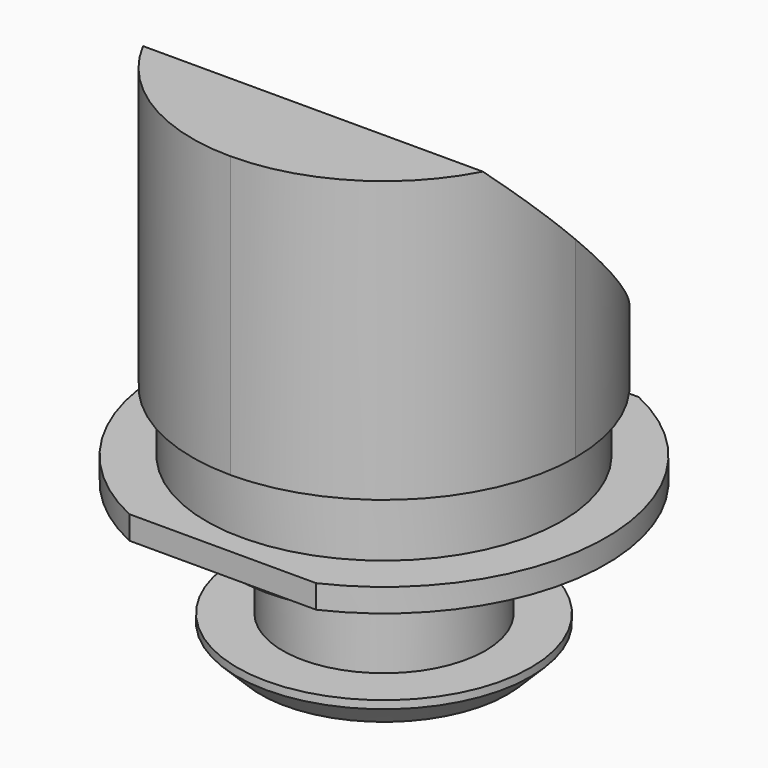
from build123d import *

# Parameters (mm, degrees)
F0_R      = 4.75
F1_DEPTH  = 0.5
F2_R      = 3.8
F3_DEPTH  = 1.3
F5_DEPTH  = 1.801
F6_R      = 3.15
F7_DEPTH  = 0.8
F8_R      = 2.165
F9_DEPTH  = 1.67
F10_R     = 3.14
F11_DEPTH = 0.67
F12_SIZE  = 0.5
F13_W     = 8.2
F13_H     = 8.2
F13_R     = 3.8
F14_DEPTH = 6
F15_SIZE  = 5.99999
F17_DEPTH = 6.001


# Not quite as in the source:
# - a fillet or chamfer is up to 0.001 mm smaller than in the source, because OpenCascade refuses the exact size


with BuildPart() as f1:
    # F0 (on Top) → F1 (new body)
    with BuildSketch(Plane.XY):
        Circle(F0_R)
    extrude(amount=F1_DEPTH)

    # F2 (on face) → F3 (join)
    with BuildSketch(Plane.XY.offset(0.5)):
        Circle(F2_R)
    extrude(amount=F3_DEPTH)

    # F4 (on face) → F5 (cut, through all)
    with BuildSketch(Plane(origin=(0, 0, 0), x_dir=(1, 0, 0), z_dir=(0, 0, -1))):
        with BuildLine():
            Line((-1.9965971051, 4.31), (0, 4.31))
            Line((0, 4.31), (1.9965971051, 4.31))
            ThreePointArc((1.9965971051, 4.31), (0, 4.75), (-1.9965971051, 4.31))
        make_face()
        with BuildLine():
            Line((0, -4.31), (-1.9965971051, -4.31))
            ThreePointArc((-1.9965971051, -4.31), (0, -4.75), (1.9965971051, -4.31))
            Line((1.9965971051, -4.31), (0, -4.31))
        make_face()
    extrude(amount=-F5_DEPTH, mode=Mode.SUBTRACT)

    # F6 (on face) → F7 (join)
    with BuildSketch(Plane(origin=(0, 0, 0), x_dir=(1, 0, 0), z_dir=(0, 0, -1))):
        Circle(F6_R)
    extrude(amount=F7_DEPTH)

    # F8 (on face) → F9 (join)
    with BuildSketch(Plane(origin=(0, 0, -0.8), x_dir=(1, 0, 0), z_dir=(0, 0, -1))):
        Circle(F8_R)
    extrude(amount=F9_DEPTH)

    # F10 (on face) → F11 (join)
    with BuildSketch(Plane(origin=(0, 0, -2.47), x_dir=(1, 0, 0), z_dir=(0, 0, -1))):
        Circle(F10_R)
    extrude(amount=F11_DEPTH)

    # F12
    f12_edges = [f1.edges().sort_by_distance(p)[0] for p in [
        (-3.14, 0, -3.14),
    ]]
    chamfer(f12_edges, length=F12_SIZE)

    # F13 (on face) → F14 (join)
    with BuildSketch(Plane.XY.offset(1.8)):
        Rectangle(F13_W, F13_H)
        Circle(F13_R, mode=Mode.SUBTRACT)
        Circle(F13_R)
    extrude(amount=F14_DEPTH)

    # F15 (size 6 in the source; OpenCascade refuses exactly that, so slightly less here)
    f15_edges = [f1.edges().sort_by_distance(p)[0] for p in [
        (0, 4.1, 7.8),
    ]]
    chamfer(f15_edges, length=F15_SIZE)

    # F16 (on face) → F17 (cut, through all)
    with BuildSketch(Plane(origin=(0, 0, 1.8), x_dir=(1, 0, 0), z_dir=(0, 0, -1))):
        with BuildLine():
            ThreePointArc((0, 4.1), (2.8991378029, 2.8991378029), (4.1, 0))
            Line((4.1, 0), (4.1, 4.1))
            Line((4.1, 4.1), (0, 4.1))
        make_face()
        with BuildLine():
            Line((4.1, -4.1), (4.1, 0))
            ThreePointArc((4.1, 0), (2.8991378029, -2.8991378029), (0, -4.1))
            Line((0, -4.1), (4.1, -4.1))
        make_face()
        with BuildLine():
            ThreePointArc((-4.1, 0), (-2.8991378029, 2.8991378029), (0, 4.1))
            Line((0, 4.1), (-4.1, 4.1))
            Line((-4.1, 4.1), (-4.1, 0))
        make_face()
        with BuildLine():
            Line((-4.1, -4.1), (0, -4.1))
            ThreePointArc((0, -4.1), (-2.8991378029, -2.8991378029), (-4.1, 0))
            Line((-4.1, 0), (-4.1, -4.1))
        make_face()
    extrude(amount=-F17_DEPTH, mode=Mode.SUBTRACT)


solid = f1.part
